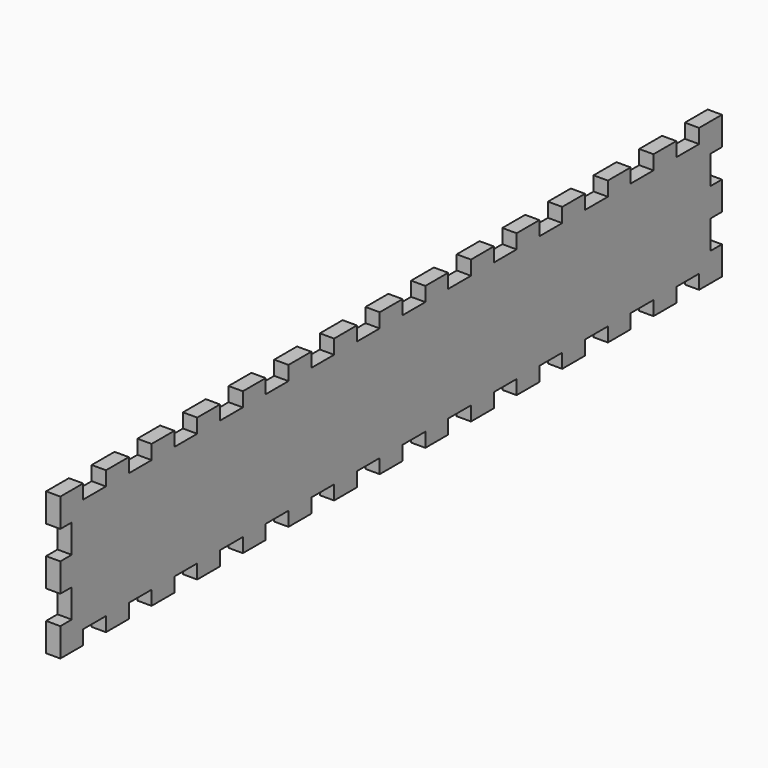
from build123d import *

# Parameters (mm, degrees)
F1_DEPTH = 2.5


# Not quite as in the source:
# - ends of sketch curves that miss each other by under 0.0002 mm in the source are joined


with BuildPart() as f1:
    # F0 (on Right) → F1 (new body, symmetric)
    with BuildSketch(Plane.YZ):
        Polygon((-135, 25), (-145, 25), (-144.9999958277, 15), (-139.9999958277, 15), (-139.9999958277, 5), (-144.9999958277, 5), (-144.9999958277, -5), (-139.9999958277, -5), (-139.9999958277, -15), (-144.9999958277, -15), (-144.9999958277, -25), (-135, -25), (-135, -20), (-125, -20), (-125, -25), (-115, -25), (-115, -20), (-105, -20), (-105, -25), (-95, -25), (-95, -20), (-85, -20), (-85, -25), (-75, -25), (-75, -20), (-65, -20), (-65, -25), (-55, -25), (-55, -20), (-45, -20), (-45, -25), (-35, -25), (-35, -20), (-25, -20), (-25, -25), (-15, -25), (-15, -20), (-5, -20), (-5, -25), (5, -25), (5, -20), (15, -20), (15, -25), (25, -25), (25, -20), (35, -20), (35, -25), (45, -25), (45, -20), (55, -20), (55, -25), (65, -25), (65, -20), (75, -20), (75, -25), (85, -25), (85, -20), (95, -20), (95, -25), (105, -25), (105, -20), (115, -20), (115, -25), (125, -25), (125, -20), (135, -20), (135, -25), (145, -25), (145, -15), (140, -15), (140, -5), (145, -5), (145, 5), (140, 5), (140, 15), (145, 15), (145, 25), (135, 25), (135, 20), (125, 20), (125, 25), (115, 25), (115, 20), (105, 20), (105, 25), (95, 25), (95, 20), (85, 20), (85, 25), (75, 25), (75, 20), (65, 20), (65, 25), (55, 25), (55, 20), (45, 20), (45, 25), (35, 25), (35, 20), (25, 20), (25, 25), (15, 25), (15, 20), (5, 20), (5, 25), (-5, 25), (-5, 20), (-15, 20), (-15, 25), (-25, 25), (-25, 20), (-35, 20), (-35, 25), (-45, 25), (-45, 20), (-55, 20), (-55, 25), (-65, 25), (-65, 20), (-75, 20), (-75, 25), (-85, 25), (-85, 20), (-95, 20), (-95, 25), (-105, 25), (-105, 20), (-115, 20), (-115, 25), (-125, 25), (-125, 20), (-135, 20), align=None)
    extrude(amount=F1_DEPTH, both=True)


solid = f1.part
